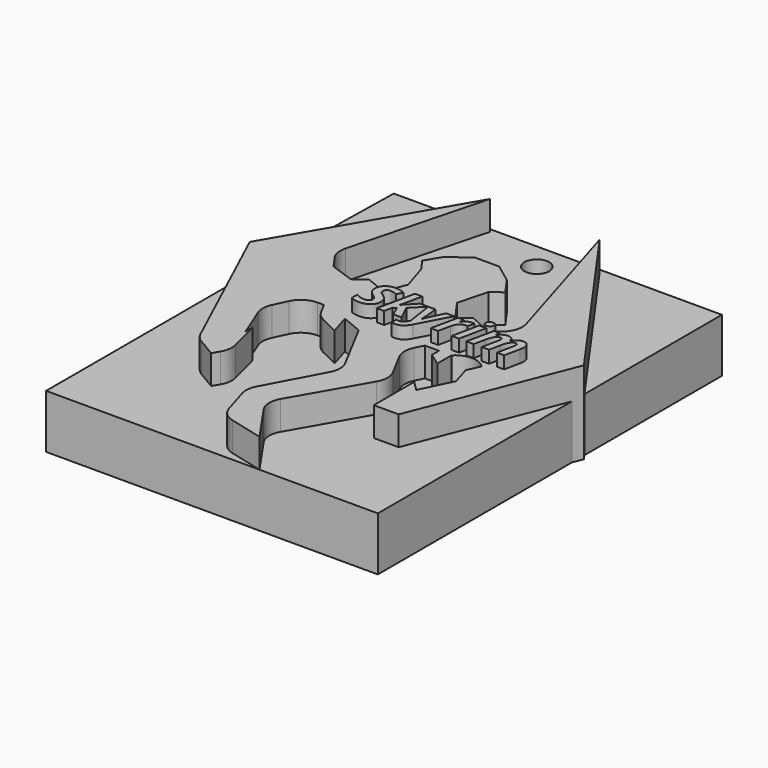
from build123d import *

# Parameters (mm, degrees)
F1_DEPTH     = 25.4
F3_DEPTH     = 16.51
F5_D         = 7.62
F6_TEXT_SIZE = 15.2540399641
F7_DEPTH     = 29.21


# Not quite as in the source:
# - Text() gives the source's letters only with a copy of the font that has no kerning and outlines rounded to 1/6400 em; it was checked with that copy


with BuildPart() as f1:
    # F0 (on Top) → F1 (new body)
    with BuildSketch(Plane.XY):
        Polygon((-20.0515763469, 2.561875576), (-23.664005175, 0), (-13.7321116854, 0), align=None)
        with BuildLine():
            Line((-13.7321116854, 0), (-23.664005175, 0))
            Line((-23.664005175, 0), (-31.0242865235, 2.561875576))
            Line((-31.0242865235, 2.561875576), (-33.7017392968, 6.3372765653))
            ThreePointArc((-33.7017392968, 6.3372765653), (-34.7700084116, 8.8767460681), (-34.6621956054, 11.6296501087))
            Line((-34.6621956054, 11.6296501087), (-23.664005175, 53.3400028944))
            Line((-23.664005175, 53.3400028944), (-54.70071733, 0))
            Line((-54.70071733, 0), (-34.0297119831, -44.7435672208))
            ThreePointArc((-34.0297119831, -44.7435672208), (-32.9787191039, -46.3353874804), (-31.5024006367, -47.5432622895))
            Line((-31.5024006367, -47.5432622895), (-25.8535724133, -50.8907139301))
            Line((-25.8535724133, -50.8907139301), (-24.6129748234, -48.7972041704))
            ThreePointArc((-24.6129748234, -48.7972041704), (-23.7902538149, -46.4622189078), (-23.9229408654, -43.9900902337))
            Line((-23.9229408654, -43.9900902337), (-26.397857815, -34.2900007963))
            Line((-26.397857815, -34.2900007963), (-26.397857815, -37.0114296675))
            Line((-26.397857815, -37.0114296675), (-30.2662841316, -27.340362405))
            ThreePointArc((-30.2662841316, -27.340362405), (-30.7173416952, -24.7831477065), (-30.1070619508, -22.2591907787))
            Line((-30.1070619508, -22.2591907787), (-28.1194644947, -18.0716305149))
            ThreePointArc((-28.1194644947, -18.0716305149), (-25.7764166039, -15.4273243108), (-22.3828595647, -14.4444716557))
            Line((-22.3828595647, -14.4444716557), (-20.3559024768, -14.4444716557))
            Line((-20.3559024768, -14.4444716557), (-18.6463269273, -17.6663652404))
            ThreePointArc((-18.6463269273, -17.6663652404), (-17.4659562036, -19.2405569729), (-15.8603681143, -20.3778526881))
            Line((-15.8603681143, -20.3778526881), (-10.0512088827, -23.2613846645))
            Line((-10.0512088827, -23.2613846645), (-11.974286288, -16.872856766))
            Line((-11.974286288, -16.872856766), (-5.6587463546, -19.4700203464))
            Line((-5.6587463546, -19.4700203464), (2.494634102, -34.8360123287))
            ThreePointArc((2.494634102, -34.8360123287), (3.2353526329, -37.8260330704), (2.4817615622, -40.8128354535))
            Line((2.4817615622, -40.8128354535), (-6.5343538385, -57.6293978665))
            ThreePointArc((-6.5343538385, -57.6293978665), (-7.2563149445, -59.9967207338), (-7.0184461681, -62.4602271457))
            Line((-7.0184461681, -62.4602271457), (-4.5723000502, -70.5864069214))
            ThreePointArc((-4.5723000502, -70.5864069214), (-2.8848185995, -73.3412505159), (-0.0602864703, -74.9092987065))
            Line((-0.0602864703, -74.9092987065), (10.3414291516, -77.5607153773))
            Line((10.3414291516, -77.5607153773), (2.2750608571, -65.8857080045))
            ThreePointArc((2.2750608571, -65.8857080045), (1.155052929, -62.5440800529), (1.9893497231, -59.1199241007))
            Line((1.9893497231, -59.1199241007), (14.3156799532, -37.6010769198))
            ThreePointArc((14.3156799532, -37.6010769198), (15.1548001768, -34.5475571789), (14.4148978226, -31.4684907516))
            Line((14.4148978226, -31.4684907516), (10.5141593465, -24.1170962634))
            ThreePointArc((10.5141593465, -24.1170962634), (9.7738904939, -21.2175484932), (10.4438138139, -18.3009446478))
            Line((10.4438138139, -18.3009446478), (11.7021435872, -15.7842859626))
            Line((11.7021435872, -15.7842859626), (16.0564277321, -15.7842859626))
            Line((16.0564277321, -15.7842859626), (16.0564277321, -18.5057139024))
            Line((16.0564277321, -18.5057139024), (19.866431132, -21.2271418422))
            Line((19.866431132, -21.2271418422), (19.866431132, -15.7842859626))
            Line((19.866431132, -15.7842859626), (20.0027308211, -15.6479862186))
            ThreePointArc((20.0027308211, -15.6479862186), (24.4928585072, -13.7881133752), (28.9829869422, -15.6479844108))
            Line((28.9829869422, -15.6479844108), (29.1192885488, -15.7842859626))
            Line((29.1192885488, -15.7842859626), (27.3383915754, -19.6652290652))
            Line((27.3383915754, -19.6652290652), (29.1192885488, -25.5814287812))
            Line((29.1192885488, -25.5814287812), (24.4928579777, -35.1064279675))
            Line((24.4928579777, -35.1064279675), (21.4992854744, -32.1128591895))
            Line((21.4992854744, -32.1128591895), (21.4992854744, -47.6250015199))
            Line((21.4992854744, -47.6250015199), (29.1192885488, -47.6250015199))
            Line((29.1192885488, -47.6250015199), (47.8971451521, 0))
            Line((47.8971451521, 0), (10.0692855194, 53.3400028944))
            Line((10.0692855194, 53.3400028944), (23.6632633845, 8.180350661))
            ThreePointArc((23.6632633845, 8.180350661), (22.6791101771, 2.561875576), (17.5827768531, 0))
            Line((17.5827768531, 0), (8.3618555973, 0))
            Line((8.3618555973, 0), (-13.7321116854, 0))
        make_face()
        Polygon((-11.1578572541, 6.35), (-13.7321116854, 0), (8.3618555973, 0), (3.8585392187, 6.35), (6.2592863105, 15.5121432617), (9.5056747814, 17.8144289896), (5.7816586595, 23.0655595757), (0, 27.3748363369), (-7.3478566483, 27.3748363369), (-13.4242468313, 23.0655595757), (-16.3285713643, 18.2335712016), (-13.7321116854, 14.572376301), align=None)
        Polygon((11.9742844254, 2.561875576), (8.3618555973, 0), (17.5827768531, 0), align=None)
    extrude(amount=F1_DEPTH)

    # F2 (on Top) → F3 (join)
    with BuildSketch(Plane.XY):
        Polygon((-54.0908239782, 54.5087531209), (-55.189114064, 0), (-55.189114064, -77.5607153773), (46.6773621738, -77.5607153773), (46.6773621738, 54.5087531209), align=None)
    extrude(amount=F3_DEPTH)

    # F5 (through all)
    with Locations(Plane(origin=(0, 0, 0), x_dir=(1, 0, 0), z_dir=(0, 0, -1))):
        with Locations((-3.5694458056, -46.2715774775)):
            Hole(F5_D / 2)

    # F6 (on Top) → F7 (join)
    with BuildSketch(Plane.XY):
        with Locations((-13.1794875488, -13.5852750391)):
            Text('Skyrim', F6_TEXT_SIZE, font='Open Sans', font_style=FontStyle.BOLDITALIC, text_align=(TextAlign.LEFT, TextAlign.BOTTOM))
    extrude(amount=F7_DEPTH)


solid = f1.part
